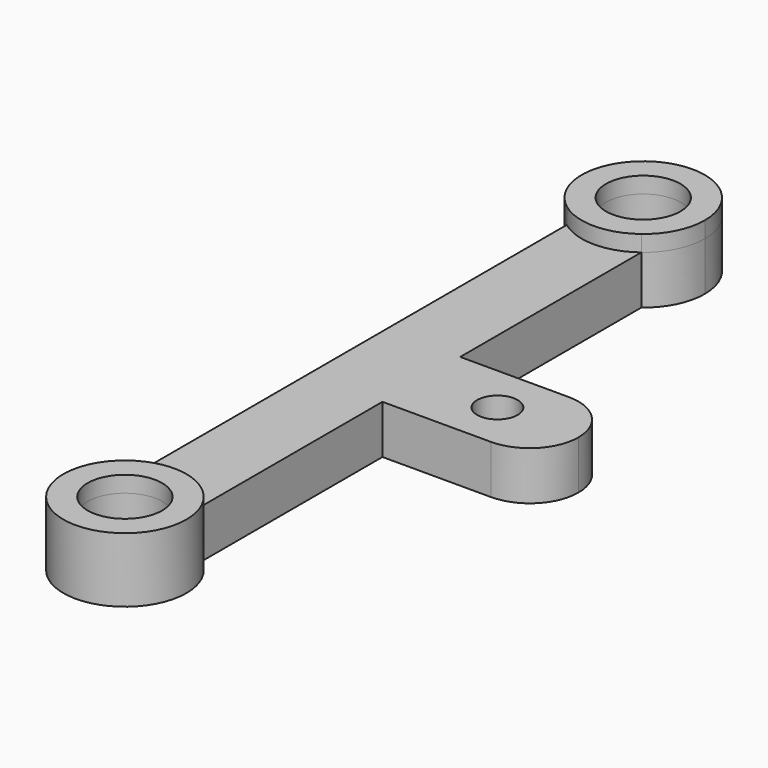
from build123d import *

# Parameters (mm, degrees)
F0_W     = 9.7
F0_H     = 6
F1_DEPTH = 3
F2_R     = 1.25
F3_DEPTH = 25
F4_R     = 2.99999
F5_R     = 2.3
F6_DEPTH = 1


# Not quite as in the source:
# - a fillet or chamfer is up to 0.001 mm smaller than in the source, because OpenCascade refuses the exact size
# - a feature names something its author has since deleted; it is built from what else it names


with BuildPart() as f1:
    # F0 (on Top) → F1 (new body)
    with BuildSketch(Plane.XY):
        with BuildLine():
            ThreePointArc((-14.3, 5), (-12, 7.3), (-9.7, 5))
            Line((-9.7, 5), (-9.7, 8.0248966925))
            ThreePointArc((-9.7, 8.0248966925), (-12, 8.8), (-14.3, 8.0248966925))
            Line((-14.3, 8.0248966925), (-14.3, 5))
        make_face()
        with BuildLine():
            Line((-9.7, 8.0248966925), (-9.7, 5))
            ThreePointArc((-9.7, 5), (-12, 2.7), (-14.3, 5))
            Line((-14.3, 5), (-14.3, 8.0248966925))
            ThreePointArc((-14.3, 8.0248966925), (-13.6881943016, 1.5955910939), (-8.2, 5))
            ThreePointArc((-8.2, 5), (-8.5955910939, 6.6881943016), (-9.7, 8.0248966925))
        make_face()
        with BuildLine():
            ThreePointArc((-8.2, 45), (-13.6881943016, 48.4044089061), (-14.3, 41.9751033075))
            Line((-14.3, 41.9751033075), (-14.3, 45))
            ThreePointArc((-14.3, 45), (-12, 47.3), (-9.7, 45))
            Line((-9.7, 45), (-9.7, 41.9751033075))
            ThreePointArc((-9.7, 41.9751033075), (-8.5955910939, 43.3118056984), (-8.2, 45))
        make_face()
        with BuildLine():
            Line((-14.3, 45), (-14.3, 41.9751033075))
            ThreePointArc((-14.3, 41.9751033075), (-12, 41.2), (-9.7, 41.9751033075))
            Line((-9.7, 41.9751033075), (-9.7, 45))
            ThreePointArc((-9.7, 45), (-12, 42.7), (-14.3, 45))
        make_face()
        with BuildLine():
            ThreePointArc((-14.3, 8.0248966925), (-12, 8.8), (-9.7, 8.0248966925))
            Line((-9.7, 8.0248966925), (-9.7, 22))
            Line((-9.7, 22), (-9.7, 28))
            Line((-9.7, 28), (-9.7, 41.9751033075))
            ThreePointArc((-9.7, 41.9751033075), (-12, 41.2), (-14.3, 41.9751033075))
            Line((-14.3, 41.9751033075), (-14.3, 8.0248966925))
        make_face()
        with Locations((-4.85, 25)):
            Rectangle(F0_W, F0_H)
        with BuildLine():
            ThreePointArc((-8.2, 45), (-13.6881943016, 48.4044089061), (-14.3, 41.9751033075))
            Line((-14.3, 41.9751033075), (-14.3, 45))
            ThreePointArc((-14.3, 45), (-12, 47.3), (-9.7, 45))
            Line((-9.7, 45), (-9.7, 41.9751033075))
            ThreePointArc((-9.7, 41.9751033075), (-8.5955910939, 43.3118056984), (-8.2, 45))
        make_face()
    extrude(amount=F1_DEPTH)

    # F2 (on face) → F3 (cut)
    with BuildSketch(Plane.XY.offset(3)):
        with Locations((-5, 25)):
            Circle(F2_R)
    extrude(amount=-F3_DEPTH, mode=Mode.SUBTRACT)

    # F4 (radius 3 in the source; OpenCascade refuses exactly that, so slightly less here)
    f4_edges = [f1.edges().sort_by_distance(p)[0] for p in [
        (0, 28, 1.5),
        (0, 22, 1.5),
    ]]
    fillet(f4_edges, radius=F4_R)

    # F5 (on face) → F6 (join)
    with BuildSketch(Plane.XY.offset(3)):
        with BuildLine():
            ThreePointArc((-14.3, 8.0248966925), (-13.6881943016, 1.5955910939), (-8.2, 5))
            ThreePointArc((-8.2, 5), (-8.5955910939, 6.6881943016), (-9.7, 8.0248966925))
            ThreePointArc((-9.7, 8.0248966925), (-12, 8.8), (-14.3, 8.0248966925))
        make_face()
        with Locations((-12, 5)):
            Circle(F5_R, mode=Mode.SUBTRACT)
        with BuildLine():
            ThreePointArc((-8.2, 45), (-13.6881943016, 48.4044089061), (-14.3, 41.9751033075))
            ThreePointArc((-14.3, 41.9751033075), (-12, 41.2), (-9.7, 41.9751033075))
            ThreePointArc((-9.7, 41.9751033075), (-8.5955910939, 43.3118056984), (-8.2, 45))
        make_face()
        with Locations((-12, 45)):
            Circle(F5_R, mode=Mode.SUBTRACT)
    extrude(amount=F6_DEPTH)


solid = f1.part
